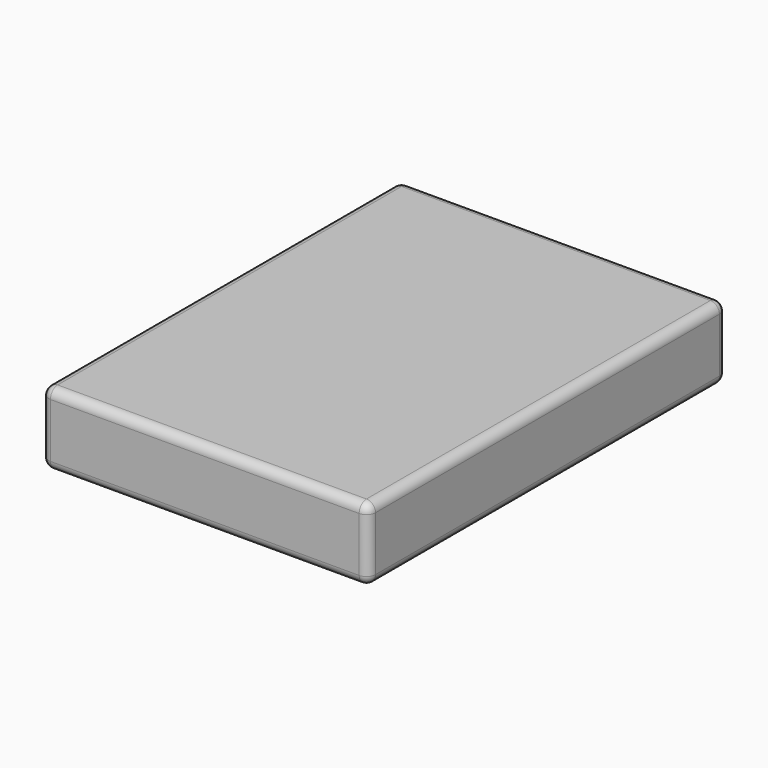
from build123d import *

# Parameters (mm, degrees)
F1_DEPTH = 1879.6
F2_R     = 38.1


with BuildPart() as f1:
    # F0 (on Front) → F1 (new body)
    with BuildSketch(Plane.XZ):
        with BuildLine():
            Line((-647.7, -152.4), (647.7, -152.4))
            ThreePointArc((647.7, -152.4), (674.6407683632, -141.2407683632), (685.8, -114.3))
            Line((685.8, -114.3), (685.8, 114.3))
            ThreePointArc((685.8, 114.3), (674.6407683632, 141.2407683632), (647.7, 152.4))
            Line((647.7, 152.4), (-647.7, 152.4))
            ThreePointArc((-647.7, 152.4), (-674.6407683632, 141.2407683632), (-685.8, 114.3))
            Line((-685.8, 114.3), (-685.8, -114.3))
            ThreePointArc((-685.8, -114.3), (-674.6407683632, -141.2407683632), (-647.7, -152.4))
        make_face()
    extrude(amount=F1_DEPTH)

    # F2
    f2_edges = [f1.edges().sort_by_distance(p)[0] for p in [
        (685.8, -1879.6, 0),
        (647.7, -939.8, 152.4),
        (685.8, 0, 0),
    ]]
    fillet(f2_edges, radius=F2_R)


solid = f1.part
